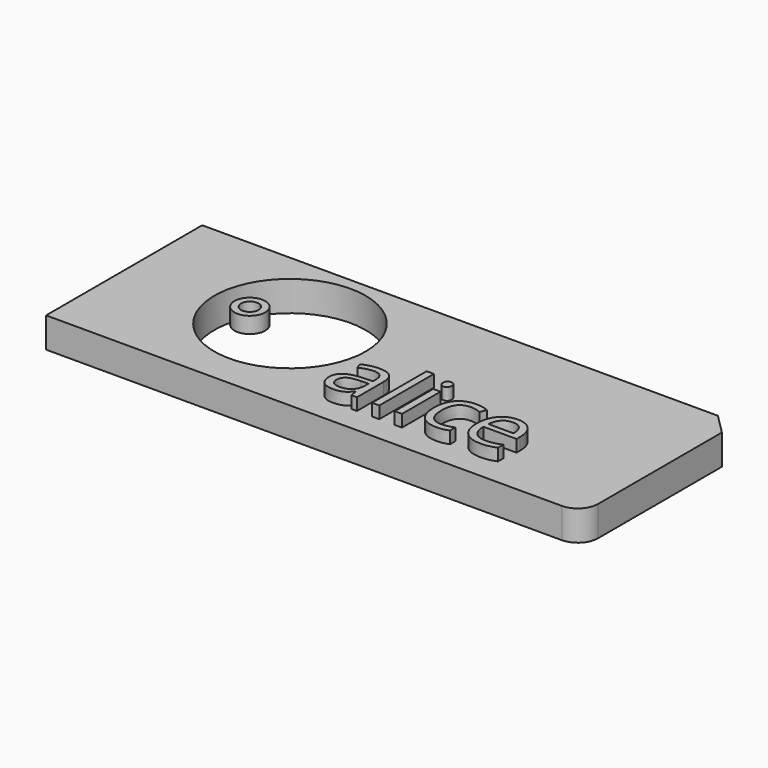
from build123d import *

# Parameters (mm, degrees)
F0_W         = 135.1815387607
F0_H         = 49.2400052026
F1_DEPTH     = 7.62
F2_R         = 19.0795455077
F3_DEPTH     = 25.4
F4_R         = 5.08
F5_SIZE      = 5.08
F6_TEXT_SIZE = 22.6926944581
F7_DEPTH     = 3.048
F8_R         = 3.8794690988
F9_DEPTH     = 4.064
F10_R        = 2.2259344521
F11_DEPTH    = 25.4


# Not quite as in the source:
# - Text() gives the source's letters only with a copy of the font that has no kerning and outlines rounded to 1/6400 em; it was checked with that copy


with BuildPart() as f1:
    # F0 (on Top) → F1 (new body)
    with BuildSketch(Plane.XY):
        with Locations((-0.2532638609, 10.5038261972)):
            Rectangle(F0_W, F0_H)
    extrude(amount=F1_DEPTH)

    # F2 (on face) → F3 (cut)
    with BuildSketch(Plane.XY.offset(7.62)):
        with Locations((-28.1263682991, 13.1530659273)):
            Circle(F2_R)
    extrude(amount=-F3_DEPTH, mode=Mode.SUBTRACT)

    # F4
    f4_edges = [f1.edges().sort_by_distance(p)[0] for p in [
        (67.337506, -14.116176, 3.81),
    ]]
    fillet(f4_edges, radius=F4_R)

    # F5
    f5_edges = [f1.edges().sort_by_distance(p)[0] for p in [
        (67.337506, 35.123829, 3.81),
    ]]
    chamfer(f5_edges, length=F5_SIZE)

    # F6 (on face) → F7 (join)
    with BuildSketch(Plane.XY.offset(7.62)):
        with Locations((-5.3222025745, -7.7018369921)):
            Text('alice', F6_TEXT_SIZE, font='Open Sans', text_align=(TextAlign.LEFT, TextAlign.BOTTOM))
    extrude(amount=F7_DEPTH)


with BuildPart() as f9:
    # F8 (on face) → F9 (new body)
    with BuildSketch(Plane.XY.offset(7.62)):
        with Locations((-33.9250378311, 7.7503393404)):
            Circle(F8_R)
    extrude(amount=F9_DEPTH)

    # F10 (on face) → F11 (cut)
    with BuildSketch(Plane.XY.offset(11.684)):
        with Locations((-33.9250378311, 7.7503393404)):
            Circle(F10_R)
    extrude(amount=-F11_DEPTH, mode=Mode.SUBTRACT)


solid = Compound([f1.part, f9.part])
